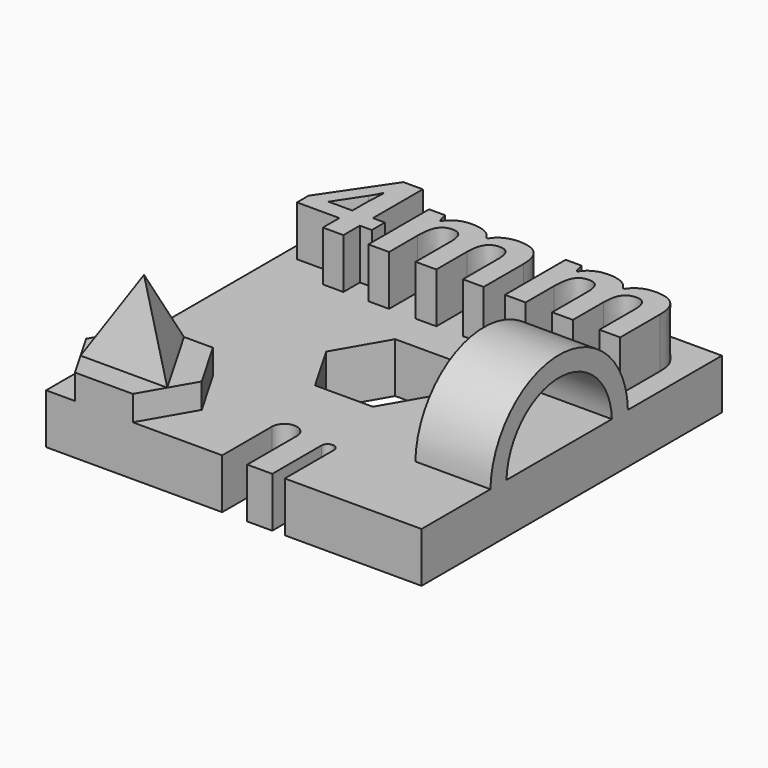
from build123d import *

# Parameters (mm, degrees)
F0_W         = 15
F0_H         = 15
F1_DEPTH     = 2
F2_TEXT_SIZE = 5.5555555556
F3_DEPTH     = 4
F5_DEPTH     = 3
F7_DEPTH     = 3
F13_DEPTH    = 2


# Not quite as in the source:
# - Text() gives the source's letters only with a copy of the font that has no kerning and outlines rounded to 1/6400 em; it was checked with that copy


with BuildPart() as f1:
    # F0 (on Top) → F1 (new body)
    with BuildSketch(Plane.XY):
        Rectangle(F0_W, F0_H)
        Polygon((-2.3094010768, 0), (-1.1547005384, 2), (1.1547005384, 2), (2.3094010768, 0), (1.1547005384, -2), (-1.1547005384, -2), align=None, mode=Mode.SUBTRACT)
    extrude(amount=F1_DEPTH)

    # F2 (on Top) → F3 (join)
    with BuildSketch(Plane.XY):
        with Locations((-7.0130208333, 3.4798150133)):
            Text('4mm', F2_TEXT_SIZE, font='Open Sans', font_style=FontStyle.BOLD, text_align=(TextAlign.LEFT, TextAlign.BOTTOM))
    extrude(amount=F3_DEPTH)

    # F4 (on Top) → F5 (join)
    with BuildSketch(Plane.XY):
        Polygon((-4.0358983849, -3.5), (-6.3452994616, -3.5), (-7.5, -5.5), (-6.3452994616, -7.5), (-4.0358983849, -7.5), (-2.8811978465, -5.5), align=None)
    extrude(amount=F5_DEPTH)

    # F6 (on face) → F7 (join)
    with BuildSketch(Plane.YZ.offset(7.5)):
        with BuildLine():
            ThreePointArc((-3.2610526842, 2), (-0.6280578673, 4.5334115069), (2.0049369496, 2))
            Line((2.0049369496, 2), (2.8053930132, 2))
            ThreePointArc((2.8053930132, 2), (-0.6280578673, 5.3334115069), (-4.0615087478, 2))
            Line((-4.0615087478, 2), (-3.2610526842, 2))
        make_face()
    extrude(amount=-F7_DEPTH)

    # F9 (on face) → F11 section 0
    with BuildSketch(Plane.XY.offset(3), mode=Mode.PRIVATE) as f11_s0:
        Polygon((-6.9226497308, -6.5), (-3.4585481157, -6.5), (-5.1905989232, -3.5), align=None)
    loft([f11_s0.sketch, Vertex(-5.1881489344, -5.4989531636, 6)])

    # F12 (on face) → F13 (cut)
    with BuildSketch(Plane.XY.offset(2)):
        with BuildLine():
            Line((-0.4642049898, -5.0183841959), (-0.4642049898, -7.5))
            Line((-0.4642049898, -7.5), (0.5357950102, -7.5))
            Line((0.5357950102, -7.5), (0.5357950102, -5.0183841959))
            ThreePointArc((0.5357950102, -5.0183841959), (0.0357950102, -4.5183841959), (-0.4642049898, -5.0183841959))
        make_face()
        with BuildLine():
            Line((1.5357950102, -5.0455084182), (1.5357950102, -7.5))
            Line((1.5357950102, -7.5), (2.0357950102, -7.5))
            Line((2.0357950102, -7.5), (2.0357950102, -5.0455084182))
            ThreePointArc((2.0357950102, -5.0455084182), (1.7857950102, -4.7955084182), (1.5357950102, -5.0455084182))
        make_face()
    extrude(amount=-F13_DEPTH, mode=Mode.SUBTRACT)


solid = f1.part
